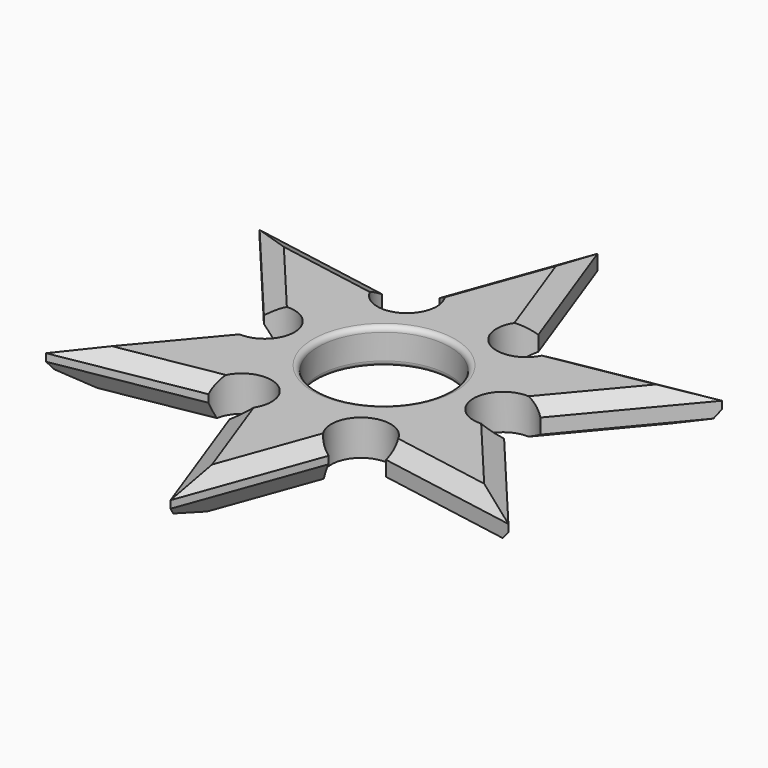
from build123d import *

# Parameters (mm, degrees)
F0_R         = 11.1
F1_DEPTH     = 6
F2_C1_SIZE2  = 3
F2_C1_SIZE   = 1.7320508076
F2_C2_SIZE2  = 3
F2_C2_SIZE   = 1.7320508076
F2_C3_SIZE2  = 3
F2_C3_SIZE   = 1.7320508076
F2_C4_SIZE2  = 3
F2_C4_SIZE   = 1.7320508076
F2_C5_SIZE2  = 1.7320508076
F2_C5_SIZE   = 3
F2_C6_SIZE2  = 3
F2_C6_SIZE   = 1.7320508076
F2_C7_SIZE2  = 1.7320508076
F2_C7_SIZE   = 3
F2_C8_SIZE2  = 3
F2_C8_SIZE   = 1.7320508076
F2_C9_SIZE2  = 1.7320508076
F2_C9_SIZE   = 3
F2_C10_SIZE2 = 3
F2_C10_SIZE  = 1.7320508076
F2_C11_SIZE2 = 3
F2_C11_SIZE  = 1.7320508076
F2_C12_SIZE2 = 3
F2_C12_SIZE  = 1.7320508076
F2_C13_SIZE2 = 1.7320508076
F2_C13_SIZE  = 3
F2_C14_SIZE2 = 3
F2_C14_SIZE  = 1.7320508076
F2_C15_SIZE2 = 3
F2_C15_SIZE  = 1.7320508076
F2_C16_SIZE2 = 3
F2_C16_SIZE  = 1.7320508076
F2_C17_SIZE2 = 1.7320508076
F2_C17_SIZE  = 3
F2_C18_SIZE2 = 3
F2_C18_SIZE  = 1.7320508076
F2_C19_SIZE2 = 3
F2_C19_SIZE  = 1.7320508076
F2_C20_SIZE2 = 3
F2_C20_SIZE  = 1.7320508076
F2_C21_SIZE2 = 1.7320508076
F2_C21_SIZE  = 3
F2_C22_SIZE2 = 3
F2_C22_SIZE  = 1.7320508076
F2_C23_SIZE2 = 3
F2_C23_SIZE  = 1.7320508076
F2_C24_SIZE2 = 3
F2_C24_SIZE  = 1.7320508076
F3_R         = 0.875


with BuildPart() as f1:
    # F0 (on Top) → F1 (new body)
    with BuildSketch(Plane.XY):
        with BuildLine():
            Line((8.3388454559, 22.1051900243), (0, 45))
            Line((0, 45), (-8.3388454559, 22.1051900243))
            ThreePointArc((-8.3388454559, 22.1051900243), (-7.55, 13.0769835971), (-14.9742333886, 18.2742470152))
            Line((-14.9742333886, 18.2742470152), (-38.9711431703, 22.5))
            Line((-38.9711431703, 22.5), (-23.3130788445, 3.8309430091))
            ThreePointArc((-23.3130788445, 3.8309430091), (-15.1, 0), (-23.3130788445, -3.8309430091))
            Line((-23.3130788445, -3.8309430091), (-38.9711431703, -22.5))
            Line((-38.9711431703, -22.5), (-14.9742333886, -18.2742470152))
            ThreePointArc((-14.9742333886, -18.2742470152), (-7.55, -13.0769835971), (-8.3388454559, -22.1051900243))
            Line((-8.3388454559, -22.1051900243), (0, -45))
            Line((0, -45), (8.3388454559, -22.1051900243))
            ThreePointArc((8.3388454559, -22.1051900243), (7.55, -13.0769835971), (14.9742333886, -18.2742470152))
            Line((14.9742333886, -18.2742470152), (38.9711431703, -22.5))
            Line((38.9711431703, -22.5), (23.3130788445, -3.8309430091))
            ThreePointArc((23.3130788445, -3.8309430091), (15.1, 0), (23.3130788445, 3.8309430091))
            Line((23.3130788445, 3.8309430091), (38.9711431703, 22.5))
            Line((38.9711431703, 22.5), (14.9742333886, 18.2742470152))
            ThreePointArc((14.9742333886, 18.2742470152), (7.55, 13.0769835971), (8.3388454559, 22.1051900243))
        make_face()
        Circle(F0_R, mode=Mode.SUBTRACT)
    extrude(amount=F1_DEPTH)

    # F2: chamfer of 3 x 1.7320508076 on 24 edges, made by hand

    # F2_c1
    f2_c1_edges = [f1.edges().sort_by_distance(p)[0] for p in [
        (31.1421110074, 13.1654715045, 0),
    ]]
    f2_c1_side = f1.faces().sort_by_distance((31.1421110074, 13.1654715045, 0.0346410162))[0]
    chamfer(f2_c1_edges, length=F2_C1_SIZE, length2=F2_C1_SIZE2, reference=f2_c1_side)

    # F2_c2
    f2_c2_edges = [f1.edges().sort_by_distance(p)[0] for p in [
        (31.1421110074, 13.1654715045, 6),
    ]]
    f2_c2_side = f1.faces().sort_by_distance((31.1421110074, 13.1654715045, 5.9653589838))[0]
    chamfer(f2_c2_edges, length=F2_C2_SIZE, length2=F2_C2_SIZE2, reference=f2_c2_side)

    # F2_c3
    f2_c3_edges = [f1.edges().sort_by_distance(p)[0] for p in [
        (24.6756919125, 19.9826322901, 0),
    ]]
    f2_c3_side = f1.faces().sort_by_distance((24.6816996097, 19.9485162005, 0))[0]
    chamfer(f2_c3_edges, length=F2_C3_SIZE, length2=F2_C3_SIZE2, reference=f2_c3_side)

    # F2_c4
    f2_c4_edges = [f1.edges().sort_by_distance(p)[0] for p in [
        (24.6756919125, 19.9826322901, 6),
    ]]
    f2_c4_side = f1.faces().sort_by_distance((24.6756919125, 19.9826322901, 5.9653589838))[0]
    chamfer(f2_c4_edges, length=F2_C4_SIZE, length2=F2_C4_SIZE2, reference=f2_c4_side)

    # F2_c5
    f2_c5_edges = [f1.edges().sort_by_distance(p)[0] for p in [
        (4.169422728, 33.5525950122, 0),
    ]]
    f2_c5_side = f1.faces().sort_by_distance((4.136873479, 33.5407397857, 0))[0]
    chamfer(f2_c5_edges, length=F2_C5_SIZE, length2=F2_C5_SIZE2, reference=f2_c5_side)

    # F2_c6
    f2_c6_edges = [f1.edges().sort_by_distance(p)[0] for p in [
        (4.169422728, 33.5525950122, 6),
    ]]
    f2_c6_side = f1.faces().sort_by_distance((4.169422728, 33.5525950122, 5.9653589838))[0]
    chamfer(f2_c6_edges, length=F2_C6_SIZE, length2=F2_C6_SIZE2, reference=f2_c6_side)

    # F2_c7
    f2_c7_edges = [f1.edges().sort_by_distance(p)[0] for p in [
        (-4.9676212415, 31.3610921973, 0),
    ]]
    f2_c7_side = f1.faces().sort_by_distance((-4.9350719925, 31.3492369708, 0))[0]
    chamfer(f2_c7_edges, length=F2_C7_SIZE, length2=F2_C7_SIZE2, reference=f2_c7_side)

    # F2_c8
    f2_c8_edges = [f1.edges().sort_by_distance(p)[0] for p in [
        (-4.9676212415, 31.3610921973, 6),
    ]]
    f2_c8_side = f1.faces().sort_by_distance((-4.9676212415, 31.3610921973, 5.9653589838))[0]
    chamfer(f2_c8_edges, length=F2_C8_SIZE, length2=F2_C8_SIZE2, reference=f2_c8_side)

    # F2_c9
    f2_c9_edges = [f1.edges().sort_by_distance(p)[0] for p in [
        (-26.9726882794, 20.3871235076, 0),
    ]]
    f2_c9_side = f1.faces().sort_by_distance((-26.9786959766, 20.353007418, 0))[0]
    chamfer(f2_c9_edges, length=F2_C9_SIZE, length2=F2_C9_SIZE2, reference=f2_c9_side)

    # F2_c10
    f2_c10_edges = [f1.edges().sort_by_distance(p)[0] for p in [
        (-26.9726882794, 20.3871235076, 6),
    ]]
    f2_c10_side = f1.faces().sort_by_distance((-26.9726882794, 20.3871235076, 5.9653589838))[0]
    chamfer(f2_c10_edges, length=F2_C10_SIZE, length2=F2_C10_SIZE2, reference=f2_c10_side)

    # F2_c11
    f2_c11_edges = [f1.edges().sort_by_distance(p)[0] for p in [
        (-29.643313154, 11.3784599071, 0),
    ]]
    f2_c11_side = f1.faces().sort_by_distance((-29.6167716023, 11.4007207704, 0))[0]
    chamfer(f2_c11_edges, length=F2_C11_SIZE, length2=F2_C11_SIZE2, reference=f2_c11_side)

    # F2_c12
    f2_c12_edges = [f1.edges().sort_by_distance(p)[0] for p in [
        (-29.643313154, 11.3784599071, 6),
    ]]
    f2_c12_side = f1.faces().sort_by_distance((-29.643313154, 11.3784599071, 5.9653589838))[0]
    chamfer(f2_c12_edges, length=F2_C12_SIZE, length2=F2_C12_SIZE2, reference=f2_c12_side)

    # F2_c13
    f2_c13_edges = [f1.edges().sort_by_distance(p)[0] for p in [
        (-31.1421110074, -13.1654715045, 0),
    ]]
    f2_c13_side = f1.faces().sort_by_distance((-31.1155694557, -13.1877323678, 0))[0]
    chamfer(f2_c13_edges, length=F2_C13_SIZE, length2=F2_C13_SIZE2, reference=f2_c13_side)

    # F2_c14
    f2_c14_edges = [f1.edges().sort_by_distance(p)[0] for p in [
        (-31.1421110074, -13.1654715045, 6),
    ]]
    f2_c14_side = f1.faces().sort_by_distance((-31.1421110074, -13.1654715045, 5.9653589838))[0]
    chamfer(f2_c14_edges, length=F2_C14_SIZE, length2=F2_C14_SIZE2, reference=f2_c14_side)

    # F2_c15
    f2_c15_edges = [f1.edges().sort_by_distance(p)[0] for p in [
        (-24.6756919125, -19.9826322901, 0),
    ]]
    f2_c15_side = f1.faces().sort_by_distance((-24.6816996097, -19.9485162005, 0))[0]
    chamfer(f2_c15_edges, length=F2_C15_SIZE, length2=F2_C15_SIZE2, reference=f2_c15_side)

    # F2_c16
    f2_c16_edges = [f1.edges().sort_by_distance(p)[0] for p in [
        (-24.6756919125, -19.9826322901, 6),
    ]]
    f2_c16_side = f1.faces().sort_by_distance((-24.6756919125, -19.9826322901, 5.9653589838))[0]
    chamfer(f2_c16_edges, length=F2_C16_SIZE, length2=F2_C16_SIZE2, reference=f2_c16_side)

    # F2_c17
    f2_c17_edges = [f1.edges().sort_by_distance(p)[0] for p in [
        (-4.169422728, -33.5525950122, 0),
    ]]
    f2_c17_side = f1.faces().sort_by_distance((-4.136873479, -33.5407397857, 0))[0]
    chamfer(f2_c17_edges, length=F2_C17_SIZE, length2=F2_C17_SIZE2, reference=f2_c17_side)

    # F2_c18
    f2_c18_edges = [f1.edges().sort_by_distance(p)[0] for p in [
        (-4.169422728, -33.5525950122, 6),
    ]]
    f2_c18_side = f1.faces().sort_by_distance((-4.169422728, -33.5525950122, 5.9653589838))[0]
    chamfer(f2_c18_edges, length=F2_C18_SIZE, length2=F2_C18_SIZE2, reference=f2_c18_side)

    # F2_c19
    f2_c19_edges = [f1.edges().sort_by_distance(p)[0] for p in [
        (4.9676212415, -31.3610921973, 0),
    ]]
    f2_c19_side = f1.faces().sort_by_distance((4.9350719925, -31.3492369708, 0))[0]
    chamfer(f2_c19_edges, length=F2_C19_SIZE, length2=F2_C19_SIZE2, reference=f2_c19_side)

    # F2_c20
    f2_c20_edges = [f1.edges().sort_by_distance(p)[0] for p in [
        (4.9676212415, -31.3610921973, 6),
    ]]
    f2_c20_side = f1.faces().sort_by_distance((4.9676212415, -31.3610921973, 5.9653589838))[0]
    chamfer(f2_c20_edges, length=F2_C20_SIZE, length2=F2_C20_SIZE2, reference=f2_c20_side)

    # F2_c21
    f2_c21_edges = [f1.edges().sort_by_distance(p)[0] for p in [
        (26.9726882794, -20.3871235076, 0),
    ]]
    f2_c21_side = f1.faces().sort_by_distance((26.9786959766, -20.353007418, 0))[0]
    chamfer(f2_c21_edges, length=F2_C21_SIZE, length2=F2_C21_SIZE2, reference=f2_c21_side)

    # F2_c22
    f2_c22_edges = [f1.edges().sort_by_distance(p)[0] for p in [
        (26.9726882794, -20.3871235076, 6),
    ]]
    f2_c22_side = f1.faces().sort_by_distance((26.9726882794, -20.3871235076, 5.9653589838))[0]
    chamfer(f2_c22_edges, length=F2_C22_SIZE, length2=F2_C22_SIZE2, reference=f2_c22_side)

    # F2_c23
    f2_c23_edges = [f1.edges().sort_by_distance(p)[0] for p in [
        (29.643313154, -11.3784599071, 0),
    ]]
    f2_c23_side = f1.faces().sort_by_distance((29.6167716023, -11.4007207704, 0))[0]
    chamfer(f2_c23_edges, length=F2_C23_SIZE, length2=F2_C23_SIZE2, reference=f2_c23_side)

    # F2_c24
    f2_c24_edges = [f1.edges().sort_by_distance(p)[0] for p in [
        (29.643313154, -11.3784599071, 6),
    ]]
    f2_c24_side = f1.faces().sort_by_distance((29.643313154, -11.3784599071, 5.9653589838))[0]
    chamfer(f2_c24_edges, length=F2_C24_SIZE, length2=F2_C24_SIZE2, reference=f2_c24_side)

    # F3
    f3_edges = [f1.edges().sort_by_distance(p)[0] for p in [
        (-11.1, 0, 0),
        (-11.1, 0, 6),
    ]]
    fillet(f3_edges, radius=F3_R)


solid = f1.part
